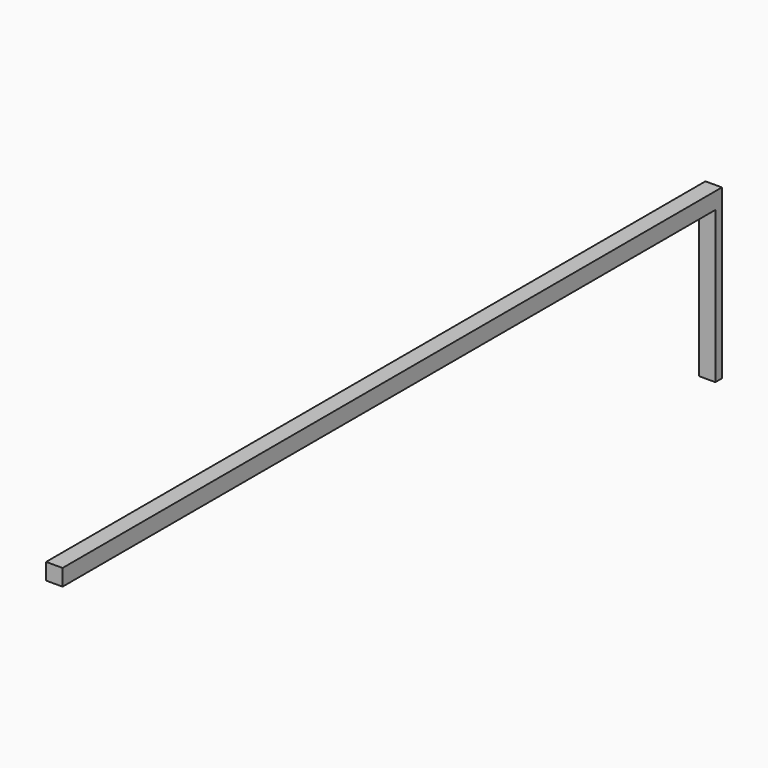
from build123d import *

# Parameters (mm, degrees)
F1_E0_W  = 92
F1_E0_H  = 10
F2_DEPTH = 5
F3_E1_W  = 500
F3_E1_H  = 10
F4_DEPTH = 10


# Not quite as in the source:
# - the program builds the solid bodies; features that only make, move or delete a surface that nothing else refers to are left out


with BuildPart() as f2:
    # F1_E0 (on explicit) → F2 (new body)
    with BuildSketch(Plane(origin=(0, 387.2919008136, 17.2254323959), x_dir=(0, 0, -1), z_dir=(0, -1, 0))):
        with Locations((46, 5)):
            Rectangle(F1_E0_W, F1_E0_H)
    extrude(amount=F2_DEPTH)

    # F3_E1 (on explicit) → F4 (join)
    with BuildSketch(Plane(origin=(0, 387.2919008136, 17.2254323959), x_dir=(0, -1, 0), z_dir=(0, 0, 1))):
        with Locations((250, 5)):
            Rectangle(F3_E1_W, F3_E1_H)
    extrude(amount=F4_DEPTH)


solid = f2.part
